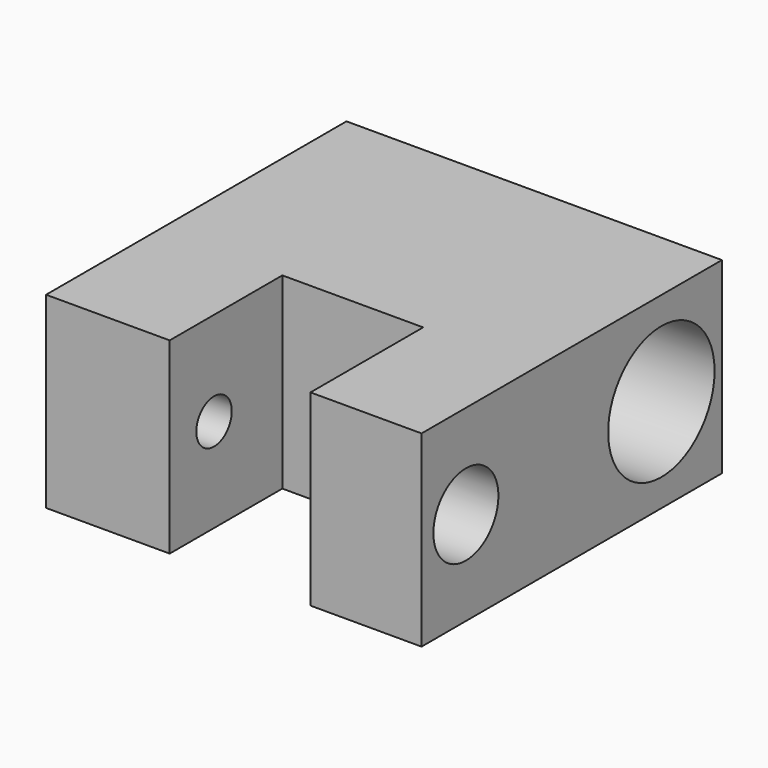
from build123d import *

# Parameters (mm, degrees)
F0_W      = 101.6
F0_H      = 101.6
F1_DEPTH  = 25.4
F2_R      = 18
F3_DEPTH  = 76.2
F4_R      = 18
F5_DEPTH  = 19.05
F6_R      = 1.5
F7_DEPTH  = 25
F8_R      = 11
F9_DEPTH  = 25.4
F10_R     = 11
F11_DEPTH = 25.4
F12_W     = 38.1
F12_H     = 43.3616997044
F13_DEPTH = 50.801
F14_R     = 6
F15_DEPTH = 76.201
F17_DEPTH = 19.05


# Not quite as in the source:
# - a length typed as a fraction of an inch, garbled in the dataset ("3 / 203.2 mm" for 3/8 in), is restored


with BuildPart() as f1:
    # F0 (on Top) → F1 (new body, symmetric)
    with BuildSketch(Plane.XY):
        with Locations((-1.7001610249, -8.4323180143)):
            Rectangle(F0_W, F0_H)
    extrude(amount=F1_DEPTH, both=True)

    # F2 (on face) → F3 (cut)
    with BuildSketch(Plane.YZ.offset(49.0998389751)):
        with Locations((21.8872688711, 0)):
            Circle(F2_R)
    extrude(amount=-F3_DEPTH, mode=Mode.SUBTRACT)

    # F4 (on face) → F5 (cut)
    with BuildSketch(Plane(origin=(-52.5001610249, 0, 0), x_dir=(0, -1, 0), z_dir=(-1, 0, 0))):
        with Locations((-21.8872688711, 0)):
            Circle(F4_R)
    extrude(amount=-F5_DEPTH, mode=Mode.SUBTRACT)

    # F6 (on face) → F7 (cut)
    with BuildSketch(Plane(origin=(-33.4501610249, 0, 0), x_dir=(0, -1, 0), z_dir=(-1, 0, 0))):
        with Locations((-21.8872688711, 0)):
            Circle(F6_R)
        with Locations((-9.838248603, 0)):
            Circle(F6_R)
        with Locations((-15.8627587371, 10.4347576428)):
            Circle(F6_R)
        with Locations((-27.9117790051, 10.4347576428)):
            Circle(F6_R)
        with Locations((-33.9362891391, 0)):
            Circle(F6_R)
        with Locations((-27.9117790051, -10.4347576428)):
            Circle(F6_R)
        with Locations((-15.8627587371, -10.4347576428)):
            Circle(F6_R)
    extrude(amount=-F7_DEPTH, mode=Mode.SUBTRACT)

    # F8 (on face) → F9 (cut)
    with BuildSketch(Plane(origin=(-52.5001610249, 0, 0), x_dir=(0, -1, 0), z_dir=(-1, 0, 0))):
        with Locations((44.2323180143, 0)):
            Circle(F8_R)
    extrude(amount=-F9_DEPTH, mode=Mode.SUBTRACT)

    # F10 (on face) → F11 (cut)
    with BuildSketch(Plane.YZ.offset(49.0998389751)):
        with Locations((-44.2323180143, 0)):
            Circle(F10_R)
    extrude(amount=-F11_DEPTH, mode=Mode.SUBTRACT)

    # F12 (on face) → F13 (cut, through all)
    with BuildSketch(Plane(origin=(0, 0, -25.4), x_dir=(1, 0, 0), z_dir=(0, 0, -1))):
        with Locations((0, 42.8131678666)):
            Rectangle(F12_W, F12_H)
    extrude(amount=-F13_DEPTH, mode=Mode.SUBTRACT)

    # F14 (on face) → F15 (cut, through all)
    with BuildSketch(Plane(origin=(-27.1001610249, 0, 0), x_dir=(0, -1, 0), z_dir=(-1, 0, 0))):
        with Locations((44.2323180143, 0)):
            Circle(F14_R)
    extrude(amount=-F15_DEPTH, mode=Mode.SUBTRACT)

    # F16 (on face) → F17 (cut)
    with BuildSketch(Plane(origin=(-52.5001610249, 0, 0), x_dir=(0, -1, 0), z_dir=(-1, 0, 0))):
        with BuildLine():
            Line((-21.8872688711, -10), (44.2323180143, -10))
            ThreePointArc((44.2323180143, -10), (54.2323180143, 0), (44.2323180143, 10))
            Line((44.2323180143, 10), (-21.8872688711, 10))
            ThreePointArc((-21.8872688711, 10), (-31.8872688711, 0), (-21.8872688711, -10))
        make_face()
    extrude(amount=-F17_DEPTH, mode=Mode.SUBTRACT)


solid = f1.part
